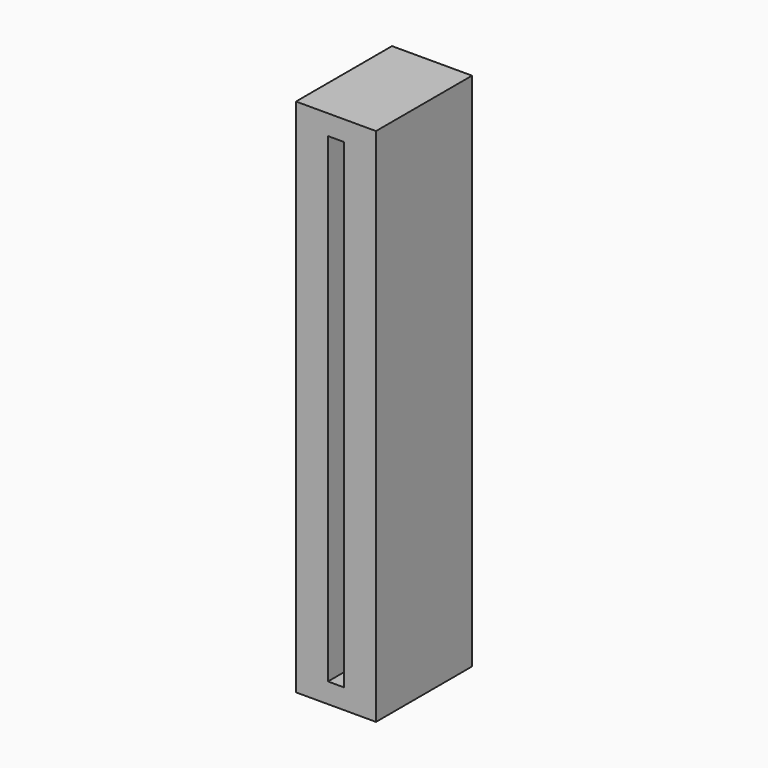
from build123d import *

# Parameters (mm, degrees)
F0_W     = 10
F0_H     = 65
F1_DEPTH = 15
F2_W     = 2
F2_H     = 60
F3_DEPTH = 10


# Not quite as in the source:
# - a feature names something its author has since deleted; it is built from what else it names


with BuildPart() as f1:
    # F0 (on Front) → F1 (new body)
    with BuildSketch(Plane.XZ):
        Rectangle(F0_W, F0_H)
    extrude(amount=F1_DEPTH)

    # F2 (on face) → F3 (cut)
    with BuildSketch(Plane.XZ.offset(15)):
        Rectangle(F2_W, F2_H)
    extrude(amount=-F3_DEPTH, mode=Mode.SUBTRACT)


solid = f1.part
